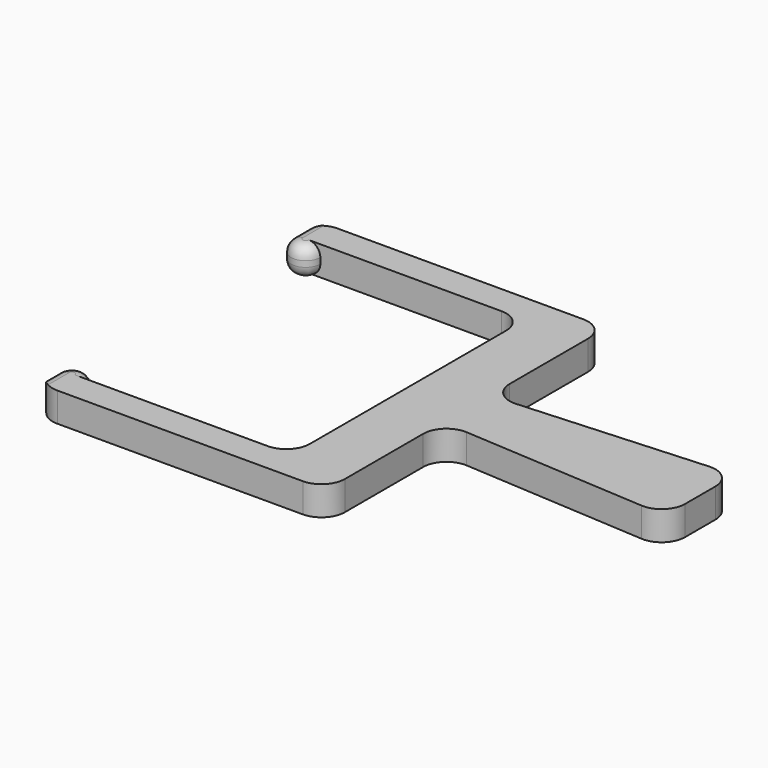
from build123d import *

# Parameters (mm, degrees)
F1_DEPTH     = 6.35
F2_F1_R      = 5.08
F2_F2_R      = 5.08
F3_T1_DEPTH  = 7.62
F3_T3_DEPTH  = 7.62
F3_T6_ANGLE  = 180
F3_T8_ANGLE  = 180
F3_T10_ANGLE = 180
F3_T12_ANGLE = 180


# Not quite as in the source:
# - a fillet or chamfer that OpenCascade refuses, or shapes differently, is made with other operations: its cross-section is extruded or revolved along the edge and cut away or added


with BuildPart() as f1:
    # F0 (on Top) → F1 (new body)
    with BuildSketch(Plane.XY):
        with BuildLine():
            Line((-31.75, -38.1), (31.75, -38.1))
            Line((31.75, -38.1), (31.75, -6.35))
            Line((31.75, -6.35), (82.55, -9.525))
            Line((82.55, -9.525), (82.55, 9.525))
            Line((82.55, 9.525), (31.75, 6.35))
            Line((31.75, 6.35), (31.75, 38.1))
            Line((31.75, 38.1), (-31.75, 38.1))
            Line((-31.75, 38.1), (-31.75, 31.75))
            ThreePointArc((-31.75, 31.75), (-28.575, 28.575), (-25.4, 31.75))
            Line((-25.4, 31.75), (19.05, 31.75))
            Line((19.05, 31.75), (19.05, -31.75))
            Line((19.05, -31.75), (-25.4, -31.75))
            ThreePointArc((-25.4, -31.75), (-28.575, -28.575), (-31.75, -31.75))
            Line((-31.75, -31.75), (-31.75, -38.1))
        make_face()
    extrude(amount=F1_DEPTH)

    # F2: fillet of radius 5.08 on 10 edges, made by hand

    # F2_f1
    f2_f1_edges = [f1.edges().sort_by_distance(p)[0] for p in [
        (19.05, -31.75, 3.175),
        (31.75, 6.35, 3.175),
        (31.75, -6.35, 3.175),
        (19.05, 31.75, 3.175),
    ]]
    fillet(f2_f1_edges, radius=F2_F1_R)

    # F2_f2
    f2_f2_edges = [f1.edges().sort_by_distance(p)[0] for p in [
        (31.75, -38.1, 3.175),
        (-31.75, -38.1, 3.175),
        (82.55, -9.525, 3.175),
        (82.55, 9.525, 3.175),
        (31.75, 38.1, 3.175),
        (-31.75, 38.1, 3.175),
    ]]
    fillet(f2_f2_edges, radius=F2_F2_R)

    # F3: fillet of radius 2.54 on 8 edges, made by hand

    # F3_s2 → F3_t1 (cut)
    with BuildSketch(Plane.XZ.offset(-39.37)):
        with BuildLine():
            ThreePointArc((-31.75, 3.81), (-31.0060512242, 5.6060512242), (-29.21, 6.35))
            Line((-29.21, 6.35), (-31.75, 6.35))
            Line((-31.75, 6.35), (-31.75, 3.81))
        make_face()
        with BuildLine():
            ThreePointArc((-29.21, 0), (-31.0060512242, 0.7439487758), (-31.75, 2.54))
            Line((-31.75, 2.54), (-31.75, 0))
            Line((-31.75, 0), (-29.21, 0))
        make_face()
    extrude(amount=F3_T1_DEPTH, mode=Mode.SUBTRACT)

    # F3_s4 → F3_t3 (cut)
    with BuildSketch(Plane.XZ.offset(31.75)):
        with BuildLine():
            ThreePointArc((-31.75, 3.81), (-31.0060512242, 5.6060512242), (-29.21, 6.35))
            Line((-29.21, 6.35), (-31.75, 6.35))
            Line((-31.75, 6.35), (-31.75, 3.81))
        make_face()
        with BuildLine():
            ThreePointArc((-29.21, 0), (-31.0060512242, 0.7439487758), (-31.75, 2.54))
            Line((-31.75, 2.54), (-31.75, 0))
            Line((-31.75, 0), (-29.21, 0))
        make_face()
    extrude(amount=F3_T3_DEPTH, mode=Mode.SUBTRACT)

    # F3_s5 → F3_t6 (revolve, cut)
    with BuildSketch(Plane.XZ.offset(-31.75)):
        with BuildLine():
            ThreePointArc((-31.75, 3.81), (-31.0060512242, 5.6060512242), (-29.21, 6.35))
            Line((-29.21, 6.35), (-31.75, 6.35))
            Line((-31.75, 6.35), (-31.75, 3.81))
        make_face()
    revolve(axis=Axis((-28.575, 31.75, 6.35), (0, 0, 1)), revolution_arc=F3_T6_ANGLE, mode=Mode.SUBTRACT)

    # F3_s7 → F3_t8 (revolve, cut)
    with BuildSketch(Plane.XZ.offset(-31.75)):
        with BuildLine():
            ThreePointArc((-29.21, 0), (-31.0060512242, 0.7439487758), (-31.75, 2.54))
            Line((-31.75, 2.54), (-31.75, 0))
            Line((-31.75, 0), (-29.21, 0))
        make_face()
    revolve(axis=Axis((-28.575, 31.75, 0), (0, 0, 1)), revolution_arc=F3_T8_ANGLE, mode=Mode.SUBTRACT)

    # F3_s9 → F3_t10 (revolve, cut)
    with BuildSketch(Plane.XZ.offset(31.75)):
        with BuildLine():
            ThreePointArc((-25.4, 3.81), (-26.1439487758, 5.6060512242), (-27.94, 6.35))
            Line((-27.94, 6.35), (-25.4, 6.35))
            Line((-25.4, 6.35), (-25.4, 3.81))
        make_face()
    revolve(axis=Axis((-28.575, -31.75, 6.35), (0, 0, 1)), revolution_arc=F3_T10_ANGLE, mode=Mode.SUBTRACT)

    # F3_s11 → F3_t12 (revolve, cut)
    with BuildSketch(Plane.XZ.offset(31.75)):
        with BuildLine():
            ThreePointArc((-27.94, 0), (-26.1439487758, 0.7439487758), (-25.4, 2.54))
            Line((-25.4, 2.54), (-25.4, 0))
            Line((-25.4, 0), (-27.94, 0))
        make_face()
    revolve(axis=Axis((-28.575, -31.75, 0), (0, 0, 1)), revolution_arc=F3_T12_ANGLE, mode=Mode.SUBTRACT)


solid = f1.part
